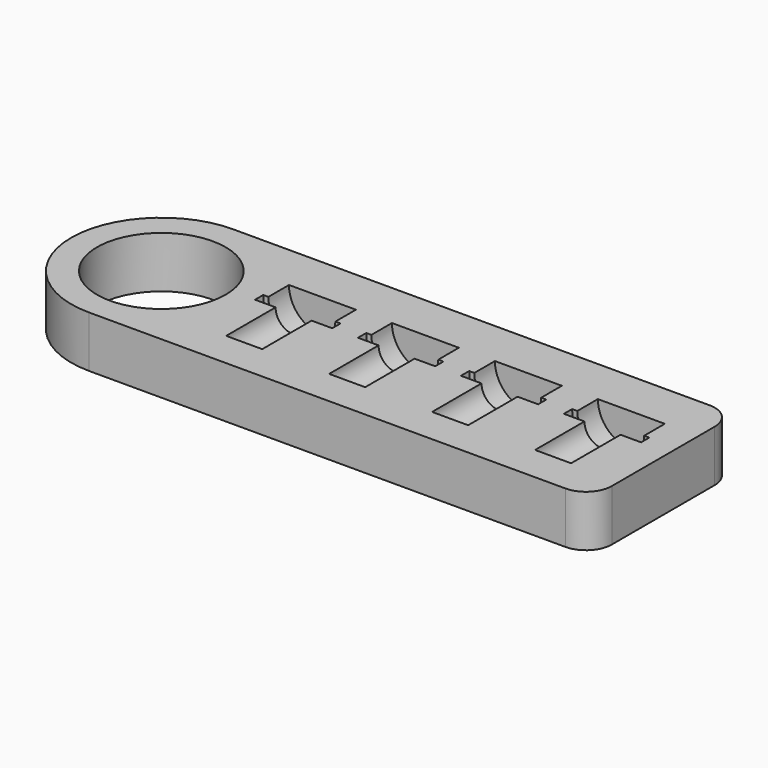
from build123d import *

# Parameters (mm, degrees)
F0_R         = 12.5
F1_DEPTH     = 10
F7_TEXT_SIZE = 5.5555555556
F8_DEPTH     = 1


# Not quite as in the source:
# - Text() gives the source's letters only with a copy of the font that has no kerning and outlines rounded to 1/6400 em; it was checked with that copy


with BuildPart() as f1:
    # F0 (on Top) → F1 (new body)
    with BuildSketch(Plane.XY):
        with BuildLine():
            ThreePointArc((0, 17.5), (5.1256313292, 5.1256313292), (17.5, 0))
            Line((17.5, 0), (110, 0))
            ThreePointArc((110, 0), (113.5355339059, 1.4644660941), (115, 5))
            Line((115, 5), (115, 30))
            ThreePointArc((115, 30), (113.5355339059, 33.5355339059), (110, 35))
            Line((110, 35), (17.5, 35))
            ThreePointArc((17.5, 35), (5.1256313292, 29.8743686708), (0, 17.5))
        make_face()
        with Locations((17.5, 17.5)):
            Circle(F0_R, mode=Mode.SUBTRACT)
    extrude(amount=F1_DEPTH)

    # F2 (on face) → F3 (revolve, cut)
    with BuildSketch(Plane.XY.offset(10)):
        Polygon((42, 19), (42, 7), (45.5, 7), (45.5, 19), (49.5, 19), (49.5, 21), (48.5, 21), (48.5, 26), (42, 26), (42, 21), align=None)
    revolve(axis=Axis((42, 23.5, 10), (0, 1, 0)), mode=Mode.SUBTRACT)

    # F2 (on face) → F4 (revolve, cut)
    with BuildSketch(Plane.XY.offset(10)):
        Polygon((62, 19), (62, 7), (65.5, 7), (65.5, 19), (69.5, 19), (69.5, 21), (68.5, 21), (68.5, 26), (62, 26), (62, 21), align=None)
    revolve(axis=Axis((62, 13, 10), (0, 1, 0)), mode=Mode.SUBTRACT)

    # F2 (on face) → F5 (revolve, cut)
    with BuildSketch(Plane.XY.offset(10)):
        Polygon((82, 19), (82, 7), (85.5, 7), (85.5, 19), (89.5, 19), (89.5, 21), (88.5, 21), (88.5, 26), (82, 26), (82, 21), align=None)
    revolve(axis=Axis((82, 13, 10), (0, 1, 0)), mode=Mode.SUBTRACT)

    # F2 (on face) → F6 (revolve, cut)
    with BuildSketch(Plane.XY.offset(10)):
        Polygon((102, 19), (102, 7), (105.5, 7), (105.5, 19), (109.5, 19), (109.5, 21), (108.5, 21), (108.5, 26), (102, 26), (102, 21), align=None)
    revolve(axis=Axis((102, 13, 10), (0, 1, 0)), mode=Mode.SUBTRACT)

    # F7 (on face) → F8 (cut)
    with BuildSketch(Plane(origin=(0, 0, 0), x_dir=(1, 0, 0), z_dir=(0, 0, -1))):
        with Locations((30, -9)):
            Text('832', F7_TEXT_SIZE, font='Open Sans', text_align=(TextAlign.LEFT, TextAlign.BOTTOM))
    extrude(amount=-F8_DEPTH, mode=Mode.SUBTRACT)


solid = f1.part
